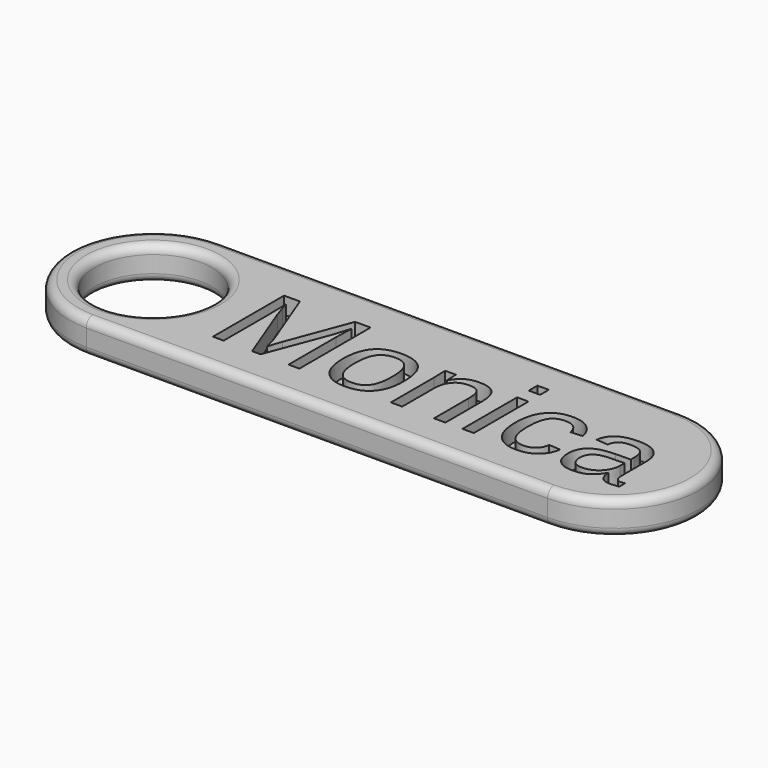
from build123d import *

# Parameters (mm, degrees)
F0_R         = 8.89
F1_DEPTH     = 5.08
F2_TEXT_SIZE = 19.5791666667
F3_DEPTH     = 2.54
F4_R         = 1.27


# Not quite as in the source:
# - Text() gives the source's letters only with a copy of the font that has no kerning and outlines rounded to 1/6400 em; it was checked with that copy


with BuildPart() as f1:
    # F0 (on Top) → F1 (new body)
    with BuildSketch(Plane.XY):
        with BuildLine():
            Line((-34.925, -12.7), (34.925, -12.7))
            ThreePointArc((34.925, -12.7), (47.625, 0), (34.925, 12.7))
            Line((34.925, 12.7), (-34.925, 12.7))
            ThreePointArc((-34.925, 12.7), (-47.625, 0), (-34.925, -12.7))
        make_face()
        with Locations((-34.925, 0)):
            Circle(F0_R, mode=Mode.SUBTRACT)
    extrude(amount=F1_DEPTH)

    # F2 (on face) → F3 (cut)
    with BuildSketch(Plane.XY.offset(5.08)):
        with Locations((-21.9255247396, -6.985)):
            Text('Monica', F2_TEXT_SIZE, font='Arimo', text_align=(TextAlign.LEFT, TextAlign.BOTTOM))
    extrude(amount=-F3_DEPTH, mode=Mode.SUBTRACT)

    # F4
    f4_edges = [f1.edges().sort_by_distance(p)[0] for p in [
        (-47.625, 0, 5.08),
        (0, -12.7, 0),
        (47.625, 0, 0),
        (0, 12.7, 0),
        (-47.625, 0, 0),
        (-43.815, 0, 0),
        (-43.815, 0, 5.08),
    ]]
    fillet(f4_edges, radius=F4_R)


solid = f1.part
